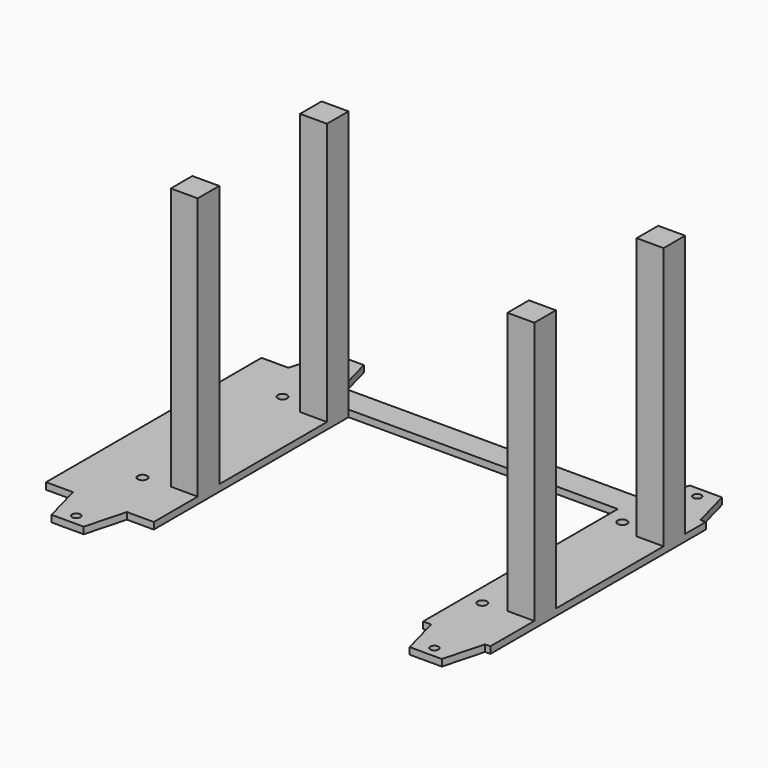
from build123d import *

# Parameters (mm, degrees)
F0_R     = 1.5
F0_R_2   = 1.75
F1_DEPTH = 2.5
F0_W     = 10
F0_H     = 10
F2_DEPTH = 100


# Not quite as in the source:
# - a feature names something its author has since deleted; it is built from what else it names


with BuildPart() as f1:
    # F0 (on Top) → F1 (new body)
    with BuildSketch(Plane.XY):
        Polygon((105.08390221, -67.8528748304), (85.08390221, -67.8528748304), (89.1031400965, -82.8528748304), (101.0646643235, -82.8528748304), align=None)
        with Locations((95.08390221, -78.8528748304)):
            Circle(F0_R, mode=Mode.SUBTRACT)
        Polygon((-47.91609779, 32.1471251696), (-57.91609779, 32.1471251696), (-57.91609779, -67.8528748304), (-47.91609779, -67.8528748304), (-27.91609779, -67.8528748304), (-17.91609779, -67.8528748304), (-17.91609779, -47.4599613249), (-27.91609779, -47.4599613249), (-27.91609779, -37.4599613249), (-17.91609779, -37.4599613249), (-17.91609779, 12.5400386751), (-27.91609779, 12.5400386751), (-27.91609779, 22.5400386751), (-17.91609779, 22.5400386751), (82.08390221, 22.5400386751), (97.08390221, 22.5400386751), (107.08390221, 22.5400386751), (107.08390221, 32.1471251696), (105.08390221, 32.1471251696), (85.08390221, 32.1471251696), (-27.91609779, 32.1471251696), align=None)
        with Locations((-37.91609779, -48.1028748304)):
            Circle(F0_R_2, mode=Mode.SUBTRACT)
        with Locations((-37.91609779, 16.8971251696)):
            Circle(F0_R_2, mode=Mode.SUBTRACT)
        Polygon((-27.91609779, -67.8528748304), (-47.91609779, -67.8528748304), (-43.8968599035, -82.8528748304), (-31.9353356765, -82.8528748304), align=None)
        with Locations((-37.91609779, -78.8528748304)):
            Circle(F0_R, mode=Mode.SUBTRACT)
        Polygon((-43.8968599035, 47.1471251696), (-47.91609779, 32.1471251696), (-27.91609779, 32.1471251696), (-31.9353356765, 47.1471251696), align=None)
        with Locations((-37.91609779, 43.1471251696)):
            Circle(F0_R, mode=Mode.SUBTRACT)
        Polygon((89.1031400965, 47.1471251696), (85.08390221, 32.1471251696), (105.08390221, 32.1471251696), (101.0646643235, 47.1471251696), align=None)
        with Locations((95.08390221, 43.1471251696)):
            Circle(F0_R, mode=Mode.SUBTRACT)
        Polygon((82.08390221, 12.5400386751), (82.08390221, -67.8528748304), (85.08390221, -67.8528748304), (105.08390221, -67.8528748304), (107.08390221, -67.8528748304), (107.08390221, -47.4599613249), (97.08390221, -47.4599613249), (97.08390221, -37.4599613249), (107.08390221, -37.4599613249), (107.08390221, 12.5400386751), (97.08390221, 12.5400386751), (97.08390221, 22.5400386751), (82.08390221, 22.5400386751), align=None)
        with Locations((88.28390221, -48.1028748304)):
            Circle(F0_R_2, mode=Mode.SUBTRACT)
        with Locations((88.28390221, 16.8971251696)):
            Circle(F0_R_2, mode=Mode.SUBTRACT)
    extrude(amount=F1_DEPTH)

    # F0 (on Top) → F2 (join)
    with BuildSketch(Plane.XY):
        with Locations((-22.91609779, 17.5400386751)):
            Rectangle(F0_W, F0_H)
        with Locations((102.08390221, 17.5400386751)):
            Rectangle(F0_W, F0_H)
        with Locations((102.08390221, -42.4599613249)):
            Rectangle(F0_W, F0_H)
        with Locations((-22.91609779, -42.4599613249)):
            Rectangle(F0_W, F0_H)
    extrude(amount=F2_DEPTH)


solid = f1.part
